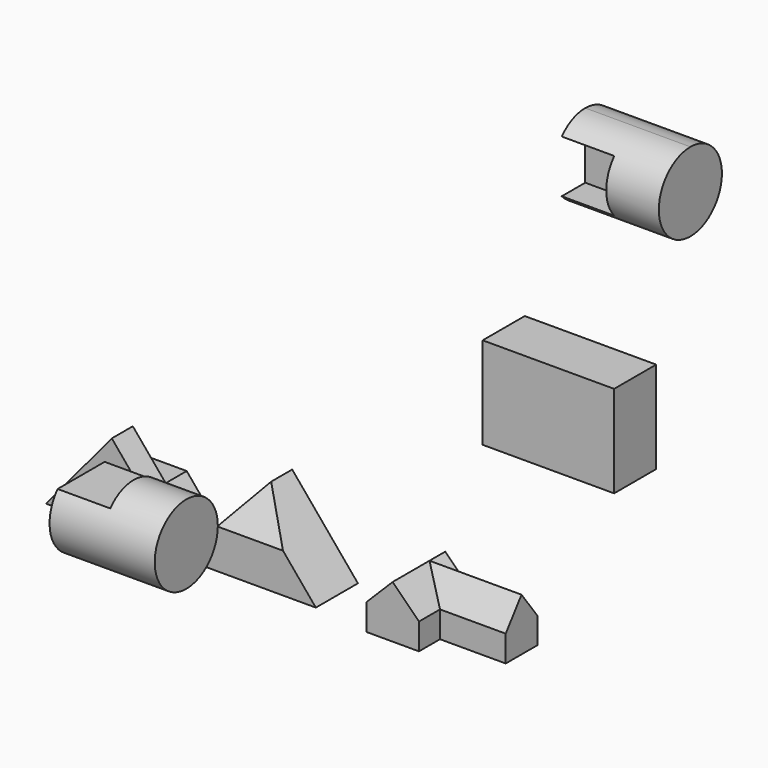
from build123d import *

# Parameters (mm, degrees)
F1_DEPTH  = 101.6
F3_DEPTH  = 50.8
F5_DEPTH  = 101.6
F9_DEPTH  = 76.2
F11_DEPTH = 127
F14_DEPTH = 177.8
F16_DEPTH = 203.2
F18_DEPTH = 101.6
F20_DEPTH = 203.2
F21_DEPTH = 101.6
F22_W     = 101.6
F22_H     = 177.8
F23_DEPTH = 254


# Not quite as in the source:
# - a feature of the source that left no trace in its solid (it failed there, or was rolled back) is left out


with BuildPart() as f1:
    # F0 (on Front) → F1 (new body)
    with BuildSketch(Plane.XZ):
        Polygon((-433.850009223, 152.4), (-560.850009223, 0), (-306.850009223, 0), align=None)
    extrude(amount=F1_DEPTH)

    # F2 (on face) → F3 (cut)
    with BuildSketch(Plane(origin=(0, 0, 0), x_dir=(-1, 0, 0), z_dir=(0, 1, 0))):
        Polygon((433.850009223, 152.4), (370.350009223, 76.2), (497.350009223, 76.2), align=None)
    extrude(amount=-F3_DEPTH, mode=Mode.SUBTRACT)


with BuildPart() as f5:
    # F4 (on Front) → F5 (new body)
    with BuildSketch(Plane.XZ):
        Polygon((-293.5190707178, -7.3142740584), (-39.5190707178, -7.3142740584), (-166.5190707178, 145.0857259416), align=None)
    extrude(amount=F5_DEPTH)

    # F8 (on 3pt) → F9 (cut, symmetric)
    with BuildSketch(Plane.YZ.offset(-166.5190707178)):
        Polygon((-50.8, 145.0857259416), (-101.6, 145.0857259416), (-101.6, 68.8857259416), align=None)
    extrude(amount=F9_DEPTH, both=True, mode=Mode.SUBTRACT)


with BuildPart() as f11:
    # F10 (on Front) → F11 (new body)
    with BuildSketch(Plane.XZ):
        Polygon((78.4911467291, 50.8), (78.4911467291, 0), (180.0911467291, 0), (180.0911467291, 50.8), (129.2911467291, 101.6), align=None)
    extrude(amount=F11_DEPTH)

    # F13 (on offset) → F14 (join)
    with BuildSketch(Plane.YZ.offset(307.0911467291)):
        Polygon((-76.2, 0), (0, 0), (0, 50.8), (-38.1, 101.6), (-76.2, 50.8), align=None)
    extrude(amount=-F14_DEPTH)


with BuildPart() as f16:
    # F15 (on Right) → F16 (new body)
    with BuildSketch(Plane.YZ):
        with BuildLine():
            ThreePointArc((-774.8033335453, 481.0394390106), (-745.1970501575, 359.0555052577), (-641.8072069168, 430.2394390106))
            ThreePointArc((-641.8072069168, 430.2394390106), (-646.8232731639, 457.4292822513), (-661.2110802883, 481.0394390106))
            Line((-661.2110802883, 481.0394390106), (-718.0072069168, 481.0394390106))
            Line((-718.0072069168, 481.0394390106), (-774.8033335453, 481.0394390106))
        make_face()
        with BuildLine():
            Line((-718.0072069168, 481.0394390106), (-661.2110802883, 481.0394390106))
            ThreePointArc((-661.2110802883, 481.0394390106), (-718.0072069168, 506.4394390106), (-774.8033335453, 481.0394390106))
            Line((-774.8033335453, 481.0394390106), (-718.0072069168, 481.0394390106))
        make_face()
    extrude(amount=F16_DEPTH)

    # F15 (on Right) → F18 (cut)
    with BuildSketch(Plane.YZ):
        with BuildLine():
            Line((-718.0072069168, 481.0394390106), (-661.2110802883, 481.0394390106))
            ThreePointArc((-661.2110802883, 481.0394390106), (-718.0072069168, 506.4394390106), (-774.8033335453, 481.0394390106))
            Line((-774.8033335453, 481.0394390106), (-718.0072069168, 481.0394390106))
        make_face()
    extrude(amount=F18_DEPTH, mode=Mode.SUBTRACT)


with BuildPart() as f20:
    # F19 (on 3pt) → F20 (new body)
    with BuildSketch(Plane.YZ.offset(-166.5190707178)):
        with BuildLine():
            Line((707.8727483749, 446.860526371), (707.8727483749, 472.260526371))
            ThreePointArc((707.8727483749, 472.260526371), (676.7642286416, 465.6212911742), (651.0766217464, 446.860526371))
            Line((651.0766217464, 446.860526371), (707.8727483749, 446.860526371))
        make_face()
        with BuildLine():
            ThreePointArc((651.0766217464, 345.260526371), (676.7642286416, 326.4997615678), (707.8727483749, 319.860526371))
            Line((707.8727483749, 319.860526371), (707.8727483749, 345.260526371))
            Line((707.8727483749, 345.260526371), (651.0766217464, 345.260526371))
        make_face()
        with BuildLine():
            ThreePointArc((707.8727483749, 319.860526371), (761.7542851014, 342.1789896446), (784.0727483749, 396.060526371))
            ThreePointArc((784.0727483749, 396.060526371), (761.7542851014, 449.9420630974), (707.8727483749, 472.260526371))
            Line((707.8727483749, 472.260526371), (707.8727483749, 446.860526371))
            Line((707.8727483749, 446.860526371), (707.8727483749, 396.060526371))
            Line((707.8727483749, 396.060526371), (707.8727483749, 345.260526371))
            Line((707.8727483749, 345.260526371), (707.8727483749, 319.860526371))
        make_face()
        with BuildLine():
            Line((707.8727483749, 446.860526371), (651.0766217464, 446.860526371))
            ThreePointArc((651.0766217464, 446.860526371), (631.6727483749, 396.060526371), (651.0766217464, 345.260526371))
            Line((651.0766217464, 345.260526371), (707.8727483749, 345.260526371))
            Line((707.8727483749, 345.260526371), (707.8727483749, 396.060526371))
            Line((707.8727483749, 396.060526371), (707.8727483749, 446.860526371))
        make_face()
    extrude(amount=F20_DEPTH)

    # F19 (on 3pt) → F21 (cut)
    with BuildSketch(Plane.YZ.offset(-166.5190707178)):
        with BuildLine():
            Line((707.8727483749, 446.860526371), (651.0766217464, 446.860526371))
            ThreePointArc((651.0766217464, 446.860526371), (631.6727483749, 396.060526371), (651.0766217464, 345.260526371))
            Line((651.0766217464, 345.260526371), (707.8727483749, 345.260526371))
            Line((707.8727483749, 345.260526371), (707.8727483749, 396.060526371))
            Line((707.8727483749, 396.060526371), (707.8727483749, 446.860526371))
        make_face()
    extrude(amount=F21_DEPTH, mode=Mode.SUBTRACT)


with BuildPart() as f23:
    # F22 (on 3pt) → F23 (new body)
    with BuildSketch(Plane.YZ.offset(-166.5190707178)):
        with Locations((510.9579086026, 88.9)):
            Rectangle(F22_W, F22_H)
    extrude(amount=F23_DEPTH)


solid = Compound([f1.part, f5.part, f11.part, f16.part, f20.part, f23.part])
